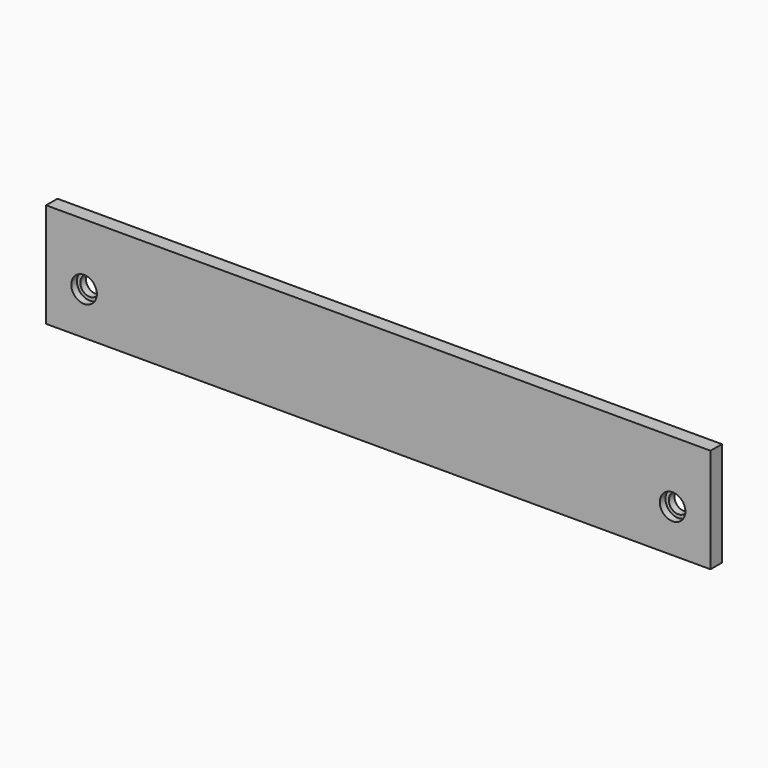
from build123d import *

# Parameters (mm, degrees)
F0_W     = 19.05
F0_H     = 139.7
F1_DEPTH = 444.5
F2_R     = 12.7
F3_DEPTH = 19.051
F4_R     = 17.145
F4_R_2   = 12.7
F5_DEPTH = 9.525


with BuildPart() as f1:
    # F0 (on Right) → F1 (new body, symmetric)
    with BuildSketch(Plane.YZ):
        Rectangle(F0_W, F0_H)
    extrude(amount=F1_DEPTH, both=True)

    # F2 (on face) → F3 (cut, through all)
    with BuildSketch(Plane.XZ.offset(9.525)):
        with Locations((-393.7, -12.7)):
            Circle(F2_R)
        with Locations((393.7, -12.7)):
            Circle(F2_R)
    extrude(amount=-F3_DEPTH, mode=Mode.SUBTRACT)

    # F4 (on face) → F5 (cut)
    with BuildSketch(Plane.XZ.offset(9.525)):
        with Locations((-393.7, -12.7)):
            Circle(F4_R)
        with Locations((-393.7, -12.7)):
            Circle(F4_R_2, mode=Mode.SUBTRACT)
        with Locations((393.7, -12.7)):
            Circle(F4_R)
        with Locations((393.7, -12.7)):
            Circle(F4_R_2, mode=Mode.SUBTRACT)
        with Locations((-393.7, -12.7)):
            Circle(F4_R_2)
    extrude(amount=-F5_DEPTH, mode=Mode.SUBTRACT)


solid = f1.part
